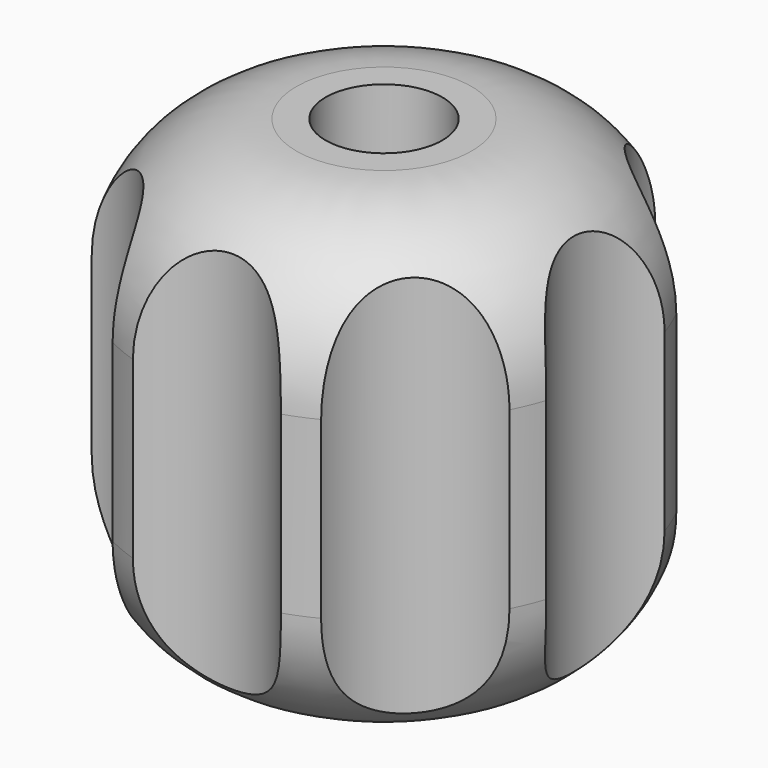
from build123d import *

# Parameters (mm, degrees)
F2_R     = 5
F3_R     = 3.5
F4_DEPTH = 25


# Not quite as in the source:
# - a feature names something its author has since deleted; it is built from what else it names


with BuildPart() as f1:
    # F0 (on Front) → F1 (revolve)
    with BuildSketch(Plane.XZ):
        Polygon((-2, 4), (-2, 16), (-8, 16), (-8, 6), (-8, 0), (0, 0), (0, 4), align=None)
    revolve(axis=Axis((0, 0, 2), (0, 0, -1)))

    # F2
    f2_edges = [f1.edges().sort_by_distance(p)[0] for p in [
        (8, 0, 0),
        (8, 0, 16),
    ]]
    fillet(f2_edges, radius=F2_R)

    # F3 (on face) → F4 (cut)
    with BuildSketch(Plane(origin=(0, 0, 0), x_dir=(1, 0, 0), z_dir=(0, 0, -1))):
        with Locations((0, 10)):
            Circle(F3_R)
        with Locations((7.0710678119, 7.0710678119)):
            Circle(F3_R)
        with Locations((10, 0)):
            Circle(F3_R)
        with Locations((7.0710678119, -7.0710678119)):
            Circle(F3_R)
        with Locations((0, -10)):
            Circle(F3_R)
        with Locations((-7.0710678119, -7.0710678119)):
            Circle(F3_R)
        with Locations((-10, 0)):
            Circle(F3_R)
        with Locations((-7.0710678119, 7.0710678119)):
            Circle(F3_R)
    extrude(amount=-F4_DEPTH, mode=Mode.SUBTRACT)


solid = f1.part
